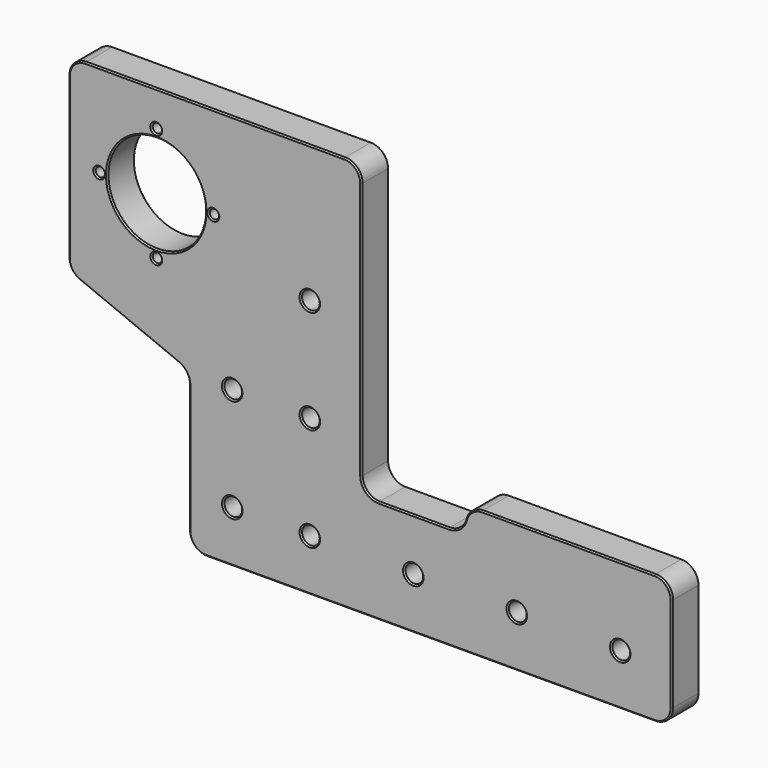
from build123d import *

# Parameters (mm, degrees)
F0_R     = 3.2639
F0_R_2   = 1.7018
F0_R_3   = 17.9959
F1_DEPTH = 12.7
F2_W     = 107.95
F2_H     = 19.2481796932
F3_DEPTH = 25.4
F4_F1_R  = 6.35
F4_F2_R  = 6.35
F5_R     = 6.35
F6_SIZE  = 0.508


with BuildPart() as f1:
    # F0 (on Front) → F1 (new body)
    with BuildSketch(Plane.XZ):
        Polygon((-126.667948618, -98.7711842824), (95.582051382, -98.4536048876), (95.582051382, -60.3536048876), (95.582051382, -50.8286048876), (19.382051382, -50.8286048876), (19.382051382, -60.3536048876), (-18.717948618, -60.3536048876), (-18.717948618, 66.3288157176), (-126.667948618, 66.3288157176), align=None)
        with Locations((-66.3308787224, -79.5945032566)):
            Circle(F0_R, mode=Mode.SUBTRACT)
        with Locations((-37.7828981478, -79.5941544378)):
            Circle(F0_R, mode=Mode.SUBTRACT)
        with Locations((-66.3853614397, -41.4661356021)):
            Circle(F0_R, mode=Mode.SUBTRACT)
        with Locations((-37.7829381848, -41.4661356021)):
            Circle(F0_R, mode=Mode.SUBTRACT)
        with Locations((0.3171018521, -79.5941544378)):
            Circle(F0_R, mode=Mode.SUBTRACT)
        with Locations((38.4171018521, -79.5941544378)):
            Circle(F0_R, mode=Mode.SUBTRACT)
        with Locations((76.5171018521, -79.5941544378)):
            Circle(F0_R, mode=Mode.SUBTRACT)
        with Locations((-117.8233242227, -10.5161073038)):
            Circle(F0_R_2, mode=Mode.SUBTRACT)
        with Locations((-94.3283242227, -8.0269073038)):
            Circle(F0_R_2, mode=Mode.SUBTRACT)
        with Locations((-115.3341242227, 12.9788926962)):
            Circle(F0_R_2, mode=Mode.SUBTRACT)
        with Locations((-94.3283242227, 12.9788926962)):
            Circle(F0_R_3, mode=Mode.SUBTRACT)
        with Locations((-73.3225242227, 12.9788926962)):
            Circle(F0_R_2, mode=Mode.SUBTRACT)
        with Locations((-70.8333242227, -10.5161073038)):
            Circle(F0_R_2, mode=Mode.SUBTRACT)
        with Locations((-37.7829381848, -3.3661356021)):
            Circle(F0_R, mode=Mode.SUBTRACT)
        with Locations((-117.8233242227, 36.4738926962)):
            Circle(F0_R_2, mode=Mode.SUBTRACT)
        with Locations((-94.3283242227, 33.9846926962)):
            Circle(F0_R_2, mode=Mode.SUBTRACT)
        with Locations((-70.8333242227, 36.4738926962)):
            Circle(F0_R_2, mode=Mode.SUBTRACT)
        with Locations((-117.8233242227, 36.4738926962)):
            Circle(F0_R_2)
        with Locations((-70.8333242227, 36.4738926962)):
            Circle(F0_R_2)
        with Locations((-70.8333242227, -10.5161073038)):
            Circle(F0_R_2)
        with Locations((-117.8233242227, -10.5161073038)):
            Circle(F0_R_2)
    extrude(amount=F1_DEPTH)

    # F2 (on face) → F3 (cut)
    with BuildSketch(Plane.XZ.offset(12.7)):
        Polygon((-82.2601616383, -40.8437248283), (-126.667948618, -22.6552803069), (-126.667948618, -98.7711842824), (-82.2601616383, -98.7077287228), align=None)
        with Locations((-72.692948618, 56.7047258711)):
            Rectangle(F2_W, F2_H)
    extrude(amount=-F3_DEPTH, mode=Mode.SUBTRACT)

    # F4: fillet of radius 6.35 on 9 edges, made by hand

    # F4_f1
    f4_f1_edges = [f1.edges().sort_by_distance(p)[0] for p in [
        (-82.2601616383, -6.35, -40.8437248283),
        (-18.717948618, -6.35, -60.3536048876),
    ]]
    fillet(f4_f1_edges, radius=F4_F1_R)

    # F4_f2
    f4_f2_edges = [f1.edges().sort_by_distance(p)[0] for p in [
        (-126.667948618, -6.35, 47.0806360245),
        (-126.667948618, -6.35, -22.6552803069),
        (-18.717948618, -6.35, 47.0806360245),
        (-82.2601616383, -6.35, -98.7077287228),
        (95.582051382, -6.35, -98.4536048876),
        (95.582051382, -6.35, -50.8286048876),
        (19.382051382, -6.35, -50.8286048876),
    ]]
    fillet(f4_f2_edges, radius=F4_F2_R)

    # F5
    f5_edges = [f1.edges().sort_by_distance(p)[0] for p in [
        (19.382051, -6.35, -60.353605),
    ]]
    fillet(f5_edges, radius=F5_R)

    # F6
    f6_edges = [f1.edges().sort_by_distance(p)[0] for p in [
        (21.843486, -12.7, -52.158489),
        (17.323894, -12.7, -59.023721),
        (57.482051, -12.7, -50.828605),
        (0.53369, -12.7, -60.353605),
        (93.722179, -12.7, -52.688477),
        (-16.858077, -12.7, -58.493733),
        (95.582051, -12.7, -74.645638),
        (-18.717949, -12.7, -6.636484),
        (93.725386, -12.7, -96.599591),
        (-20.577821, -12.7, 45.220764),
        (6.670019, -12.7, -98.580654),
        (-72.692949, -12.7, 47.080636),
        (-80.397081, -12.7, -96.841983),
        (-124.808077, -12.7, 45.220764),
        (-82.260162, -12.7, -68.726767),
        (-126.667949, -12.7, 11.168258),
        (-83.337331, -12.7, -41.566558),
        (-125.590779, -12.7, -21.932447),
        (-104.464055, -12.7, -31.749503),
        (-69.594779, -12.7, -79.594503),
        (-41.046798, -12.7, -79.594154),
        (-69.649261, -12.7, -41.466136),
        (-41.046838, -12.7, -41.466136),
        (-2.946798, -12.7, -79.594154),
        (35.153202, -12.7, -79.594154),
        (73.253202, -12.7, -79.594154),
        (-96.030124, -12.7, -8.026907),
        (-41.046838, -12.7, -3.366136),
        (-117.035924, -12.7, 12.978893),
        (-112.324224, -12.7, 12.978893),
        (-75.024324, -12.7, 12.978893),
        (-96.030124, -12.7, 33.984693),
        (21.843486, 0, -52.158489),
        (17.323894, 0, -59.023721),
        (57.482051, 0, -50.828605),
        (0.53369, 0, -60.353605),
        (93.722179, 0, -52.688477),
        (-16.858077, 0, -58.493733),
        (95.582051, 0, -74.645638),
        (-18.717949, 0, -6.636484),
        (93.725386, 0, -96.599591),
        (-20.577821, 0, 45.220764),
        (6.670019, 0, -98.580654),
        (-72.692949, 0, 47.080636),
        (-80.397081, 0, -96.841983),
        (-124.808077, 0, 45.220764),
        (-82.260162, 0, -68.726767),
        (-126.667949, 0, 11.168258),
        (-83.337331, 0, -41.566558),
        (-125.590779, 0, -21.932447),
        (-104.464055, 0, -31.749503),
        (-69.594779, 0, -79.594503),
        (-41.046798, 0, -79.594154),
        (-69.649261, 0, -41.466136),
        (-41.046838, 0, -41.466136),
        (-2.946798, 0, -79.594154),
        (35.153202, 0, -79.594154),
        (73.253202, 0, -79.594154),
        (-96.030124, 0, -8.026907),
        (-41.046838, 0, -3.366136),
        (-117.035924, 0, 12.978893),
        (-112.324224, 0, 12.978893),
        (-75.024324, 0, 12.978893),
        (-96.030124, 0, 33.984693),
    ]]
    chamfer(f6_edges, length=F6_SIZE)


solid = f1.part
